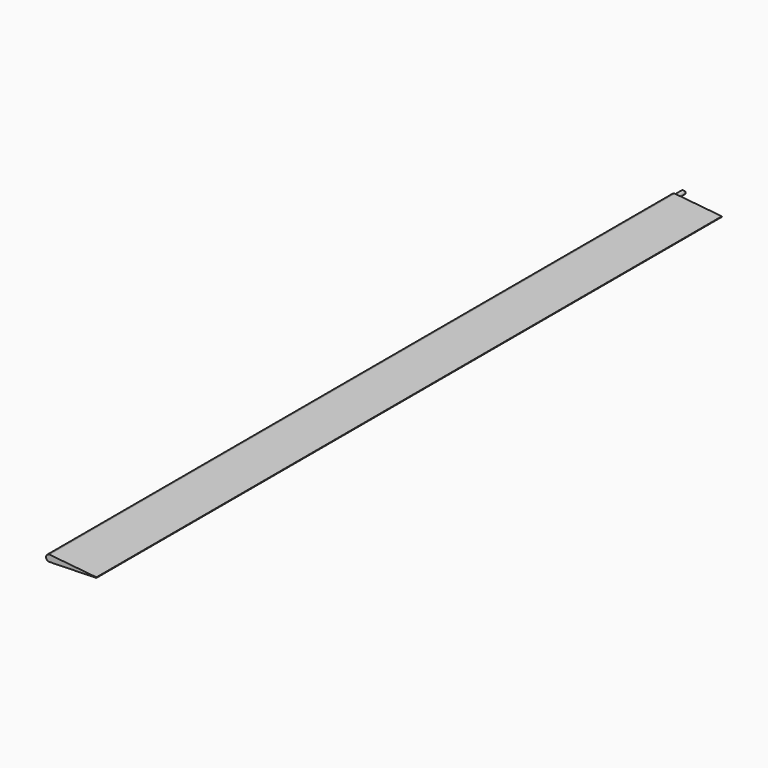
from build123d import *

# Parameters (mm, degrees)
F1_DEPTH    = 12000
F2_T1_DEPTH = 12030.8724111993
F2_T3_DEPTH = 12007.7249640069
F3_R        = 5
F4_R        = 30
F5_DEPTH    = 200
F7_DEPTH    = 50


# Not quite as in the source:
# - a fillet or chamfer that OpenCascade refuses, or shapes differently, is made with other operations: its cross-section is extruded or revolved along the edge and cut away or added


with BuildPart() as f1:
    # F0 (on Front) → F1 (new body)
    with BuildSketch(Plane.XZ):
        with BuildLine():
            Line((0, -30), (0, 50))
            ThreePointArc((0, 50), (-50, 0), (0, -50))
            Line((0, -50), (0, -30))
        make_face()
        Polygon((800, -30), (0, 50), (0, -30), align=None)
        Polygon((800, -30), (0, -30), (0, -50), align=None)
    extrude(amount=F1_DEPTH)

    # F2: fillet of radius 40 on 2 edges, made by hand

    # F2_s2 → F2_t1 (cut)
    with BuildSketch(Plane.XZ.offset(-15.4362055996)):
        with BuildLine():
            ThreePointArc((2.7476085346, 49.7252391465), (-1.7105207108, 49.9208956194), (-6.1627011311, 49.6187576907))
            ThreePointArc((-6.1627011311, 49.6187576907), (-3.0872411199, 49.904598408), (0, 50))
            Line((0, 50), (2.7476085346, 49.7252391465))
        make_face()
    extrude(amount=F2_T1_DEPTH, mode=Mode.SUBTRACT)

    # F2_s4 → F2_t3 (cut)
    with BuildSketch(Plane.XZ.offset(-3.8624820034)):
        with BuildLine():
            ThreePointArc((-1.5448083953, -49.9761299724), (-0.4270873442, -49.9950515732), (0.6907259674, -49.9827318508))
            Line((0.6907259674, -49.9827318508), (0, -50))
            ThreePointArc((0, -50), (-0.7724964007, -49.994032137), (-1.5448083953, -49.9761299724))
        make_face()
    extrude(amount=F2_T3_DEPTH, mode=Mode.SUBTRACT)

    # F3
    f3_edges = [f1.edges().sort_by_distance(p)[0] for p in [
        (800, -6000, -30),
    ]]
    fillet(f3_edges, radius=F3_R)

    # F4 (on Front) → F5 (join)
    with BuildSketch(Plane.XZ):
        Circle(F4_R)
    extrude(amount=-F5_DEPTH)

    # F6 (on Top) → F7 (cut, symmetric)
    with BuildSketch(Plane.XY):
        with BuildLine():
            ThreePointArc((0, 160), (28.2842712475, 171.7157287525), (40, 200))
            ThreePointArc((40, 200), (-28.2842712475, 228.2842712475), (0, 160))
        make_face()
    extrude(amount=F7_DEPTH, both=True, mode=Mode.SUBTRACT)


solid = f1.part
